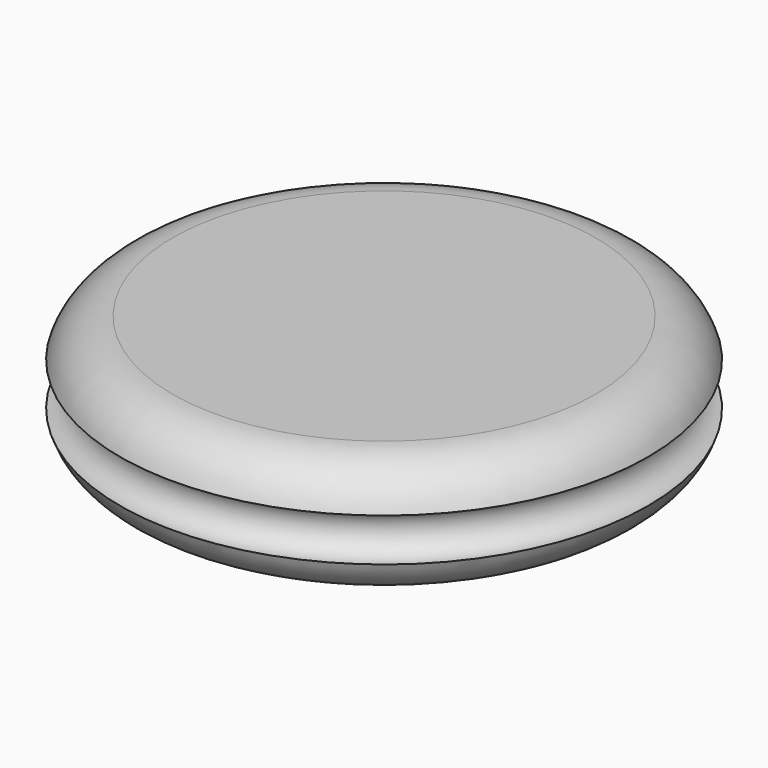
from build123d import *


# Not quite as in the source:
# - a fillet or chamfer that OpenCascade refuses, or shapes differently, is made with other operations: its cross-section is extruded or revolved along the edge and cut away or added


with BuildPart() as f1:
    # F0 (on Front) → F1 (revolve)
    with BuildSketch(Plane.XZ):
        with BuildLine():
            Line((24.442197755, 0), (0, 0))
            Line((0, 0), (0, -11.0753690824))
            Line((0, -11.0753690824), (24.442197755, -11.0753690824))
            Line((24.442197755, -11.0753690824), (24.442197755, -7.5315845412))
            ThreePointArc((24.442197755, -7.5315845412), (22.448297755, -5.5376845412), (24.442197755, -3.5437845412))
            Line((24.442197755, -3.5437845412), (24.442197755, 0))
        make_face()
    revolve(axis=Axis((0, 0, -5.5376845412), (0, 0, -1)))

    # F2: fillet of radius 5.08 on 2 edges, made by hand

    # F2_s1 → F2_t2 (revolve, cut)
    with BuildSketch(Plane.XZ):
        with BuildLine():
            ThreePointArc((24.442197755, -3.5437845412), (22.6002472435, -0.9805869609), (19.6000451279, 0))
            Line((19.6000451279, 0), (24.442197755, 0))
            Line((24.442197755, 0), (24.442197755, -3.5437845412))
        make_face()
    revolve(axis=Axis((0, 0, 0), (0, 0, -1)), mode=Mode.SUBTRACT)

    # F2_s3 → F2_t4 (revolve, cut)
    with BuildSketch(Plane.XZ):
        with BuildLine():
            ThreePointArc((19.6000451279, -11.0753690824), (22.6002472435, -10.0947821215), (24.442197755, -7.5315845412))
            Line((24.442197755, -7.5315845412), (24.442197755, -11.0753690824))
            Line((24.442197755, -11.0753690824), (19.6000451279, -11.0753690824))
        make_face()
    revolve(axis=Axis((0, 0, -11.0753690824), (0, 0, -1)), mode=Mode.SUBTRACT)


solid = f1.part
